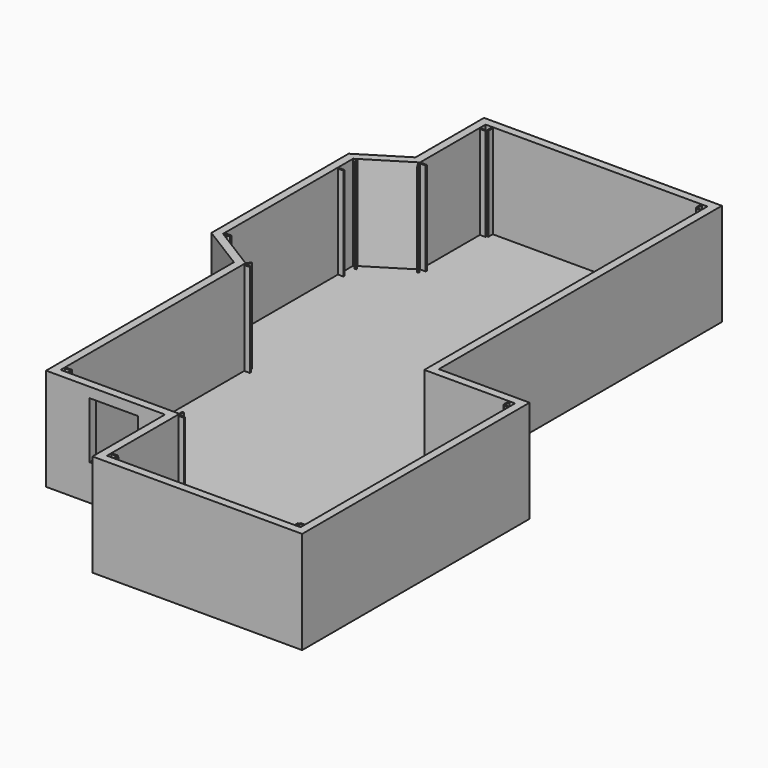
from build123d import *

# Parameters (mm, degrees)
F1_DEPTH = 2578.1
F2_T     = -203.2
F3_W     = 1219.2
F3_H     = 1422.4
F5_DEPTH = 203.2
F4_W     = 139.7
F4_H     = 38.1
F6_DEPTH = 2349.5
F4_W_2   = 38.1
F4_H_2   = 139.7


# Not quite as in the source:
# - a feature of the source that left no trace in its solid (it failed there, or was rolled back) is left out


with BuildPart() as f1:
    # F0 (on Top) → F1 (new body)
    with BuildSketch(Plane.XY):
        Polygon((-2286, 16078.2), (-8280.4, 16078.2), (-8280.4, 13922.375), (-9406.501324312, 13223.08125), (-9406.501324312, 8900.31875), (-8280.4, 8201.025), (-8280.4, 2286), (-5283.2, 2286), (-5283.2, 0), (0, 0), (0, 7162.8), (-2286, 7162.8), align=None)
    extrude(amount=F1_DEPTH)

    # F2
    f2_openings = [f1.faces().sort_by_distance(p)[0] for p in [
        (-4762.628229, 7961.579676, 2578.1),
    ]]
    offset(amount=F2_T, openings=f2_openings, kind=Kind.INTERSECTION)

    # F3 (on face) → F5 (cut, through all)
    with BuildSketch(Plane(origin=(0, 2489.2, 0), x_dir=(-1, 0, 0), z_dir=(0, 1, 0))):
        with Locations((6578.6, 1612.9)):
            Rectangle(F3_W, F3_H)
    extrude(amount=-F5_DEPTH, mode=Mode.SUBTRACT)


with BuildPart() as f6:
    # F4 (on face) → F6 (new body)
    with BuildSketch(Plane.XY.offset(203.2)):
        with Locations((-8007.35, 13830.9575758433)):
            Rectangle(F4_W, F4_H)
    extrude(amount=F6_DEPTH)


with BuildPart() as f6b:
    # F4 (on face) → F6, piece 2 (new body)
    with BuildSketch(Plane.XY.offset(203.2)):
        with Locations((-7915.91, 15805.15)):
            Rectangle(F4_W_2, F4_H_2)
    extrude(amount=F6_DEPTH)


with BuildPart() as f6c:
    # F4 (on face) → F6, piece 3 (new body)
    with BuildSketch(Plane.XY.offset(203.2)):
        with Locations((-8007.35, 15713.71)):
            Rectangle(F4_W, F4_H)
    extrude(amount=F6_DEPTH)


with BuildPart() as f6d:
    # F4 (on face) → F6, piece 4 (new body)
    with BuildSketch(Plane.XY.offset(203.2)):
        with Locations((-2650.49, 15805.15)):
            Rectangle(F4_W_2, F4_H_2)
    extrude(amount=F6_DEPTH)


with BuildPart() as f6e:
    # F4 (on face) → F6, piece 5 (new body)
    with BuildSketch(Plane.XY.offset(203.2)):
        with Locations((-2559.05, 15713.71)):
            Rectangle(F4_W, F4_H)
    extrude(amount=F6_DEPTH)


with BuildPart() as f6f:
    # F4 (on face) → F6, piece 6 (new body)
    with BuildSketch(Plane.XY.offset(203.2)):
        Polygon((-8004.5214391422, 13690.0555610339), (-8078.2194630943, 13808.7345029973), (-8110.5864472661, 13788.6350419195), (-8036.888423314, 13669.9560999561), align=None)
    extrude(amount=F6_DEPTH)


with BuildPart() as f6g:
    # F4 (on face) → F6, piece 7 (new body)
    with BuildSketch(Plane.XY.offset(203.2)):
        with Locations((-9133.451324312, 12650.4205444336)):
            Rectangle(F4_W, F4_H)
    extrude(amount=F6_DEPTH)


with BuildPart() as f6h:
    # F4 (on face) → F6, piece 8 (new body)
    with BuildSketch(Plane.XY.offset(203.2)):
        Polygon((-9129.9361601891, 13155.6326042864), (-9162.303144361, 13135.5331432085), (-9088.6051204089, 13016.8542012451), (-9056.238136237, 13036.9536623229), align=None)
    extrude(amount=F6_DEPTH)


with BuildPart() as f6i:
    # F4 (on face) → F6, piece 9 (new body)
    with BuildSketch(Plane.XY.offset(203.2)):
        Polygon((-9116.524441526, 9061.5861741567), (-9162.303144361, 8987.8668567915), (-9129.9361601891, 8967.7673957136), (-9071.6759628326, 9061.5861741567), align=None)
        Polygon((-9203.301324312, 9061.5861741567), (-9116.524441526, 9061.5861741567), (-9092.864854862, 9099.6861741567), (-9203.301324312, 9099.6861741567), align=None)
        Polygon((-9092.864854862, 9099.6861741567), (-9116.524441526, 9061.5861741567), (-9071.6759628326, 9061.5861741567), (-9063.601324312, 9074.5890947912), (-9063.601324312, 9091.0187782645), (-9077.5587863837, 9099.6861741567), align=None)
        Polygon((-9088.6051204089, 9106.5457987549), (-9092.864854862, 9099.6861741567), (-9077.5587863837, 9099.6861741567), align=None)
        Polygon((-9063.601324312, 9074.5890947912), (-9071.6759628326, 9061.5861741567), (-9063.601324312, 9061.5861741567), align=None)
        Polygon((-9063.601324312, 9099.6861741567), (-9077.5587863837, 9099.6861741567), (-9063.601324312, 9091.0187782645), align=None)
        Polygon((-9063.601324312, 9091.0187782645), (-9063.601324312, 9074.5890947912), (-9056.238136237, 9086.446337677), align=None)
    extrude(amount=F6_DEPTH)


with BuildPart() as f6j:
    # F4 (on face) → F6, piece 10 (new body)
    with BuildSketch(Plane.XY.offset(203.2)):
        Polygon((-8035.8689602197, 8452.810827198), (-8109.5669841718, 8334.1318852346), (-8077.2, 8314.0324241568), (-8003.5019760479, 8432.7113661202), align=None)
    extrude(amount=F6_DEPTH)


with BuildPart() as f6k:
    # F4 (on face) → F6, piece 11 (new body)
    with BuildSketch(Plane.XY.offset(203.2)):
        with Locations((-8007.35, 8292.4424241568)):
            Rectangle(F4_W, F4_H)
    extrude(amount=F6_DEPTH)


with BuildPart() as f6l:
    # F4 (on face) → F6, piece 12 (new body)
    with BuildSketch(Plane.XY.offset(203.2)):
        with Locations((-8007.35, 2650.49)):
            Rectangle(F4_W, F4_H)
    extrude(amount=F6_DEPTH)


with BuildPart() as f6m:
    # F4 (on face) → F6, piece 13 (new body)
    with BuildSketch(Plane.XY.offset(203.2)):
        with Locations((-7915.91, 2559.05)):
            Rectangle(F4_W_2, F4_H_2)
    extrude(amount=F6_DEPTH)


with BuildPart() as f6n:
    # F4 (on face) → F6, piece 14 (new body)
    with BuildSketch(Plane.XY.offset(203.2)):
        with Locations((-5101.59, 2559.05)):
            Rectangle(F4_W_2, F4_H_2)
    extrude(amount=F6_DEPTH)


with BuildPart() as f6o:
    # F4 (on face) → F6, piece 15 (new body)
    with BuildSketch(Plane.XY.offset(203.2)):
        with Locations((-5010.15, 2467.61)):
            Rectangle(F4_W, F4_H)
    extrude(amount=F6_DEPTH)


with BuildPart() as f6p:
    # F4 (on face) → F6, piece 16 (new body)
    with BuildSketch(Plane.XY.offset(203.2)):
        with Locations((-5010.15, 364.49)):
            Rectangle(F4_W, F4_H)
    extrude(amount=F6_DEPTH)


with BuildPart() as f6q:
    # F4 (on face) → F6, piece 17 (new body)
    with BuildSketch(Plane.XY.offset(203.2)):
        with Locations((-4918.71, 273.05)):
            Rectangle(F4_W_2, F4_H_2)
    extrude(amount=F6_DEPTH)


with BuildPart() as f6r:
    # F4 (on face) → F6, piece 18 (new body)
    with BuildSketch(Plane.XY.offset(203.2)):
        with Locations((-364.49, 273.05)):
            Rectangle(F4_W_2, F4_H_2)
    extrude(amount=F6_DEPTH)


with BuildPart() as f6s:
    # F4 (on face) → F6, piece 19 (new body)
    with BuildSketch(Plane.XY.offset(203.2)):
        with Locations((-273.05, 364.49)):
            Rectangle(F4_W, F4_H)
    extrude(amount=F6_DEPTH)


with BuildPart() as f6t:
    # F4 (on face) → F6, piece 20 (new body)
    with BuildSketch(Plane.XY.offset(203.2)):
        with Locations((-273.05, 6798.31)):
            Rectangle(F4_W, F4_H)
    extrude(amount=F6_DEPTH)


with BuildPart() as f6u:
    # F4 (on face) → F6, piece 21 (new body)
    with BuildSketch(Plane.XY.offset(203.2)):
        with Locations((-364.49, 6889.75)):
            Rectangle(F4_W_2, F4_H_2)
    extrude(amount=F6_DEPTH)


solid = Compound([f1.part, f6.part, f6b.part, f6c.part, f6d.part, f6e.part, f6f.part, f6g.part, f6h.part, f6i.part, f6j.part, f6k.part, f6l.part, f6m.part, f6n.part, f6o.part, f6p.part, f6q.part, f6r.part, f6s.part, f6t.part, f6u.part])
